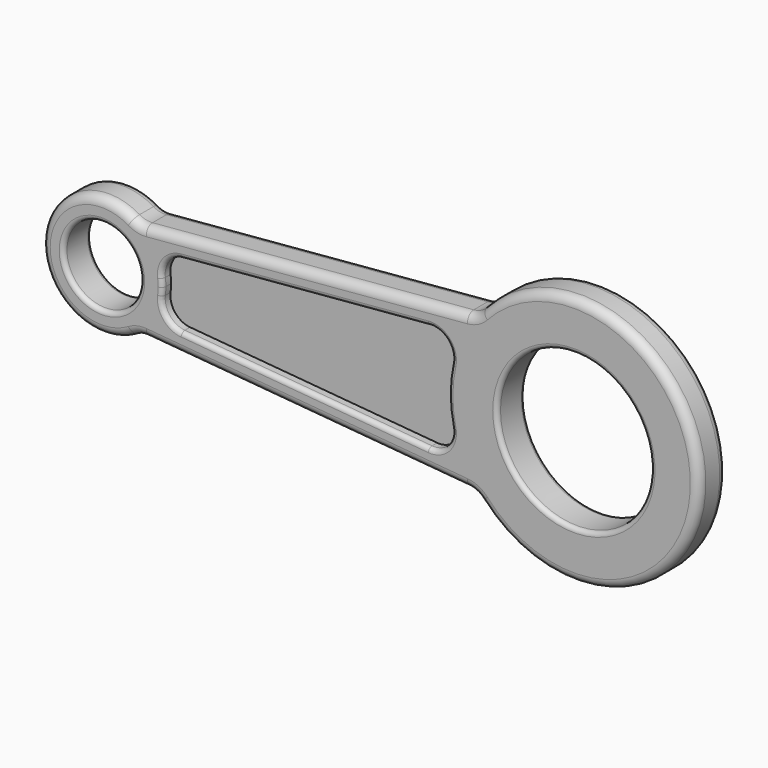
from build123d import *

# Parameters (mm, degrees)
F0_R     = 8.89
F1_DEPTH = 4
F3_DEPTH = 27.8
F4_R     = 4.99999
F5_R     = 4.99999
F6_R     = 5
F7_R     = 2
F9_DEPTH = 1.5
F10_R    = 1
F11_R    = 1


# Not quite as in the source:
# - a fillet or chamfer is up to 0.001 mm smaller than in the source, because OpenCascade refuses the exact size


with BuildPart() as f1:
    # F0 (on Front) → F1 (new body, symmetric)
    with BuildSketch(Plane.XZ):
        with BuildLine():
            ThreePointArc((8.368879315, -11.1858284901), (12.491479977, -6.2549043146), (13.97, 0))
            ThreePointArc((13.97, 0), (12.491479977, 6.2549043146), (8.368879315, 11.1858284901))
            ThreePointArc((8.368879315, 11.1858284901), (-13.97, 0), (8.368879315, -11.1858284901))
        make_face()
        Circle(F0_R, mode=Mode.SUBTRACT)
        with BuildLine():
            ThreePointArc((86.4925555891, 17.9419398769), (81.865422537, 9.4961585822), (80.264, 0))
            ThreePointArc((80.264, 0), (81.865422537, -9.4961585822), (86.4925555891, -17.9419398769))
            ThreePointArc((86.4925555891, -17.9419398769), (118.7161585822, -27.354577463), (138.176, 0))
            ThreePointArc((138.176, 0), (118.7161585822, 27.354577463), (86.4925555891, 17.9419398769))
        make_face()
        with BuildLine():
            ThreePointArc((127, 0), (109.22, -17.78), (91.44, 0))
            ThreePointArc((91.44, 0), (109.22, 17.78), (127, 0))
        make_face(mode=Mode.SUBTRACT)
        with BuildLine():
            ThreePointArc((8.368879315, 11.1858284901), (12.491479977, 6.2549043146), (13.97, 0))
            Line((13.97, 0), (80.264, 0))
            ThreePointArc((80.264, 0), (81.865422537, 9.4961585822), (86.4925555891, 17.9419398769))
            Line((86.4925555891, 17.9419398769), (8.368879315, 11.1858284901))
        make_face()
        with BuildLine():
            Line((80.264, 0), (13.97, 0))
            ThreePointArc((13.97, 0), (12.491479977, -6.2549043146), (8.368879315, -11.1858284901))
            Line((8.368879315, -11.1858284901), (86.4925555891, -17.9419398769))
            ThreePointArc((86.4925555891, -17.9419398769), (81.865422537, -9.4961585822), (80.264, 0))
        make_face()
    extrude(amount=F1_DEPTH, both=True)

    # F2 (on face) → F3 (cut)
    with BuildSketch(Plane.XZ.offset(4)):
        with BuildLine():
            ThreePointArc((13.0215256718, 5.141971332), (13.7532061608, 2.6171206119), (14, 0))
            ThreePointArc((14, 0), (13.7532061608, -2.6171206119), (13.0215256718, -5.141971332))
            ThreePointArc((13.0215256718, -5.141971332), (14.6307425402, -6.6534677385), (16.734022008, -7.3245979767))
            Line((16.734022008, -7.3245979767), (77.9088617217, -12.6149792143))
            ThreePointArc((77.9088617217, -12.6149792143), (80.3313341789, -12.2197688718), (82.2738460349, -10.7193650227))
            ThreePointArc((82.2738460349, -10.7193650227), (80.22, 0), (82.2738460349, 10.7193650227))
            ThreePointArc((82.2738460349, 10.7193650227), (80.3313341789, 12.2197688718), (77.9088617217, 12.6149792143))
            Line((77.9088617217, 12.6149792143), (16.734022008, 7.3245979767))
            ThreePointArc((16.734022008, 7.3245979767), (14.6307425402, 6.6534677385), (13.0215256718, 5.141971332))
        make_face()
    extrude(amount=-F3_DEPTH, mode=Mode.SUBTRACT)

    # F4 (radius 5 in the source; OpenCascade refuses exactly that, so slightly less here)
    f4_edges = [f1.edges().sort_by_distance(p)[0] for p in [
        (13.021526, 0, -5.141971),
        (13.021526, 0, 5.141971),
    ]]
    fillet(f4_edges, radius=F4_R)

    # F5 (radius 5 in the source; OpenCascade refuses exactly that, so slightly less here)
    f5_edges = [f1.edges().sort_by_distance(p)[0] for p in [
        (82.273846, 0, -10.719365),
        (82.273846, 0, 10.719365),
    ]]
    fillet(f5_edges, radius=F5_R)

    # F6
    f6_edges = [f1.edges().sort_by_distance(p)[0] for p in [
        (8.368879, 0, 11.185828),
        (8.368879, 0, -11.185828),
        (86.492556, 0, -17.94194),
        (86.492556, 0, 17.94194),
    ]]
    fillet(f6_edges, radius=F6_R)

    # F7
    f7_edges = [f1.edges().sort_by_distance(p)[0] for p in [
        (-13.97, -4, 0),
        (-13.97, 4, 0),
    ]]
    fillet(f7_edges, radius=F7_R)

    # F8 (on Front) → F9 (join, symmetric)
    with BuildSketch(Plane.XZ):
        Polygon((83.9080438018, 15.045507811), (10.4572921991, 8.714444004), (10.4572921991, -8.7100788951), (83.9080438018, -14.7079853341), align=None)
    extrude(amount=F9_DEPTH, both=True)

    # F10
    f10_edges = [f1.edges().sort_by_distance(p)[0] for p in [
        (14, -4, 0),
        (14.937926, -4, 5.61852),
        (47.008864, -4, 9.942757),
        (14, 4, 0),
    ]]
    fillet(f10_edges, radius=F10_R)

    # F11
    f11_edges = [f1.edges().sort_by_distance(p)[0] for p in [
        (-8.89, -4, 0),
        (-8.89, 4, 0),
        (127, -4, 0),
        (127, 4, 0),
    ]]
    fillet(f11_edges, radius=F11_R)


solid = f1.part
